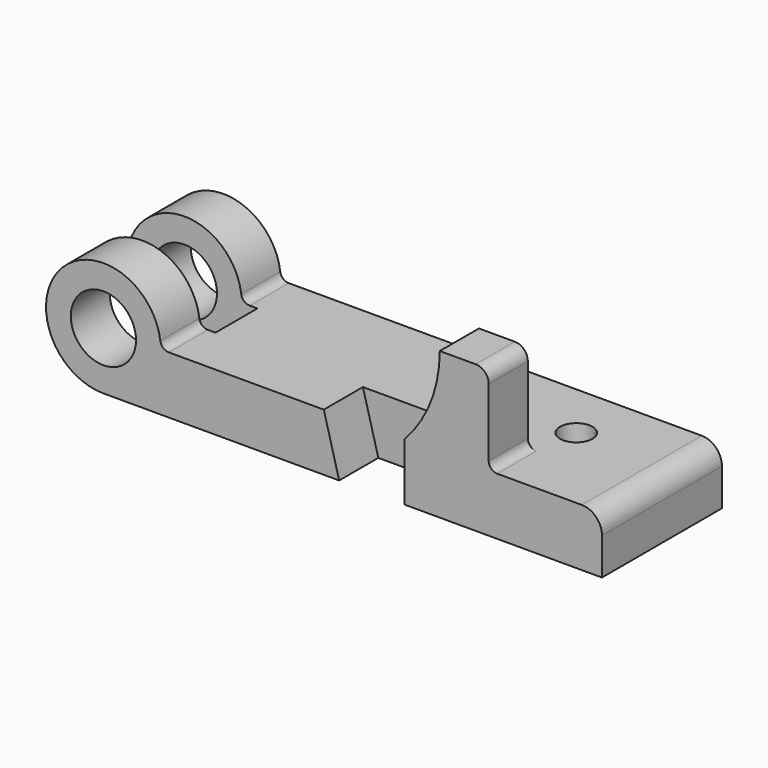
from build123d import *

# Parameters (mm, degrees)
F0_R     = 12.7
F1_DEPTH = 58.42
F2_DEPTH = 19.05
F3_DEPTH = 19.05
F4_R     = 6.35
F5_DEPTH = 38.1
F6_R     = 3.302
F7_R     = 5.08
F8_R     = 7.874
F4_W     = 44.704
F4_H     = 20.4216
F4_W_2   = 6.096
F9_DEPTH = 38.1


# Not quite as in the source:
# - a feature names something its author has since deleted; it is built from what else it names


with BuildPart() as f1:
    # F0 (on Front) → F1 (new body)
    with BuildSketch(Plane.XZ):
        Polygon((85.852, 22.352), (91.8464, 0), (117.2464, 0), (117.2464, 22.352), align=None)
        with BuildLine():
            ThreePointArc((22.352, 22.352), (15.8052507731, 6.5467492269), (0, 0))
            Line((0, 0), (91.8464, 0))
            Line((91.8464, 0), (85.852, 22.352))
            Line((85.852, 22.352), (22.352, 22.352))
        make_face()
        Polygon((117.2464, 22.352), (117.2464, 0), (194.2084, 0), (194.2084, 22.352), (150.0886, 22.352), align=None)
        with BuildLine():
            ThreePointArc((22.352, 22.352), (-15.8052507731, 38.1572507731), (0, 0))
            ThreePointArc((0, 0), (15.8052507731, 6.5467492269), (22.352, 22.352))
        make_face()
        with Locations((0, 22.352)):
            Circle(F0_R, mode=Mode.SUBTRACT)
    extrude(amount=-F1_DEPTH)

    # F0 (on Front) → F2 (cut)
    with BuildSketch(Plane.XZ):
        Polygon((85.852, 22.352), (91.8464, 0), (117.2464, 0), (117.2464, 22.352), align=None)
    extrude(amount=-F2_DEPTH, mode=Mode.SUBTRACT)

    # F0 (on Front) → F3 (join)
    with BuildSketch(Plane.XZ):
        with BuildLine():
            ThreePointArc((131.0386, 57.15), (127.4644153616, 38.4343576341), (117.2464, 22.352))
            Line((117.2464, 22.352), (150.0886, 22.352))
            Line((150.0886, 22.352), (150.0886, 57.15))
            Line((150.0886, 57.15), (131.0386, 57.15))
        make_face()
    extrude(amount=-F3_DEPTH)

    # F4 (on face) → F5 (cut, symmetric)
    with BuildSketch(Plane.XY.offset(22.352)):
        with Locations((155.3464, 36.068)):
            Circle(F4_R)
    extrude(amount=F5_DEPTH, both=True, mode=Mode.SUBTRACT)

    # F6
    f6_edges = [f1.edges().sort_by_distance(p)[0] for p in [
        (22.352, 29.21, 22.352),
        (150.0886, 9.525, 22.352),
    ]]
    fillet(f6_edges, radius=F6_R)

    # F7
    f7_edges = [f1.edges().sort_by_distance(p)[0] for p in [
        (150.0886, 9.525, 57.15),
    ]]
    fillet(f7_edges, radius=F7_R)

    # F8
    f8_edges = [f1.edges().sort_by_distance(p)[0] for p in [
        (194.2084, 29.21, 22.352),
    ]]
    fillet(f8_edges, radius=F8_R)

    # F4 (on face) → F9 (cut, symmetric)
    with BuildSketch(Plane.XY.offset(22.352)):
        with Locations((0, 29.21)):
            Rectangle(F4_W, F4_H)
        with Locations((25.4, 29.21)):
            Rectangle(F4_W_2, F4_H)
        with Locations((155.3464, 36.068)):
            Circle(F4_R)
    extrude(amount=F9_DEPTH, both=True, mode=Mode.SUBTRACT)


solid = f1.part
